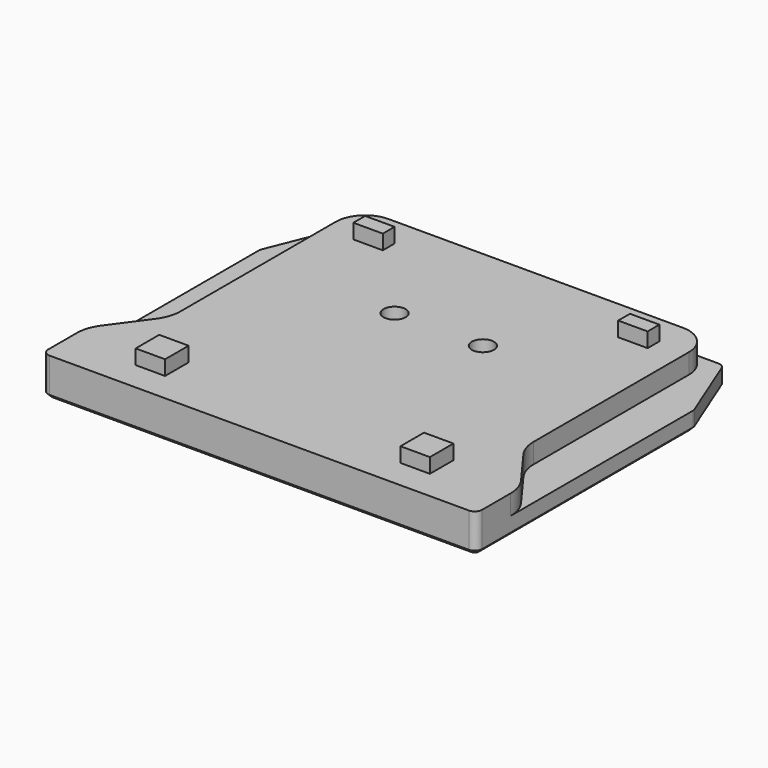
from build123d import *

# Parameters (mm, degrees)
F1_DEPTH      = 2.5
F3_DEPTH      = 2.7
F4_R          = 1
F5_R          = 5
F6_W          = 4
F6_H          = 2
F6_H_2        = 4
F7_DEPTH      = 2
F8_R          = 1.5
F9_DEPTH      = 6
F10_R         = 2.5
F11_DEPTH     = 3.5
F12_S5_R      = 1.5
F12_T6_DEPTH  = 5
F12_S11_R     = 1.5
F12_T12_DEPTH = 5
F13_SIZE      = 0.5


# Not quite as in the source:
# - a fillet or chamfer that OpenCascade refuses, or shapes differently, is made with other operations: its cross-section is extruded or revolved along the edge and cut away or added


with BuildPart() as f1:
    # F0 (on Top) → F1 (new body)
    with BuildSketch(Plane.XY):
        Polygon((55, 0), (4, 0), (0, -10), (0, -47), (59, -47), (59, -10), align=None)
    extrude(amount=F1_DEPTH)

    # F2 (on face) → F3 (join)
    with BuildSketch(Plane.XY.offset(2.5)):
        with BuildLine():
            Line((0, -39.5), (0, -47))
            Line((0, -47), (59, -47))
            Line((59, -47), (59, -39.5))
            Line((59, -39.5), (53.5, -32))
            Line((53.5, -32), (53.5, -4))
            ThreePointArc((53.5, -4), (52.3284271247, -1.1715728753), (49.5, 0))
            Line((49.5, 0), (9.5, 0))
            ThreePointArc((9.5, 0), (6.6715728753, -1.1715728753), (5.5, -4))
            Line((5.5, -4), (5.5, -32))
            Line((5.5, -32), (0, -39.5))
        make_face()
    extrude(amount=F3_DEPTH)

    # F4
    f4_edges = [f1.edges().sort_by_distance(p)[0] for p in [
        (0, -47, 2.6),
        (59, -47, 2.6),
        (4, 0, 1.25),
        (55, 0, 1.25),
        (59, -10, 1.25),
        (0, -10, 1.25),
    ]]
    fillet(f4_edges, radius=F4_R)

    # F5
    f5_edges = [f1.edges().sort_by_distance(p)[0] for p in [
        (0, -39.5, 3.85),
        (59, -39.5, 3.85),
        (53.5, -32, 3.85),
        (5.5, -32, 3.85),
    ]]
    fillet(f5_edges, radius=F5_R)

    # F6 (on face) → F7 (join)
    with BuildSketch(Plane.XY.offset(5.2)):
        with Locations((11.5, -5)):
            Rectangle(F6_W, F6_H)
        with Locations((11.5, -41)):
            Rectangle(F6_W, F6_H_2)
        with Locations((47.5, -5)):
            Rectangle(F6_W, F6_H)
        with Locations((47.5, -41)):
            Rectangle(F6_W, F6_H_2)
    extrude(amount=F7_DEPTH)

    # F8 (on face) → F9 (cut)
    with BuildSketch(Plane.XY.offset(5.2)):
        with Locations((23.5, -16.5)):
            Circle(F8_R)
        with Locations((35.5, -16.5)):
            Circle(F8_R)
    extrude(amount=-F9_DEPTH, mode=Mode.SUBTRACT)

    # F10 (on face) → F11 (cut)
    with BuildSketch(Plane.XY):
        with Locations((35.5, -16.5)):
            Circle(F10_R)
        with Locations((23.5, -16.5)):
            Circle(F10_R)
    extrude(amount=F11_DEPTH, mode=Mode.SUBTRACT)

    # F12: chamfer of 1.2 on 2 edges, made by hand


with BuildPart() as f12_tool2:
    # F12_s3 → F12_t4 (revolve)
    with BuildSketch(Plane.XZ.offset(16.5)):
        Polygon((38, 2.3), (36.8, 3.5), (38, 3.5), align=None)
    revolve(axis=Axis((35.5, -16.5, 3.5), (0, 0, 1)))

    # F12_s5 → F12_t6 (cut, symmetric)
    with BuildSketch(Plane.XY.offset(2.9)):
        with Locations((35.5, -16.5)):
            Circle(F12_S5_R)
    extrude(amount=F12_T6_DEPTH, both=True, mode=Mode.SUBTRACT)


with BuildPart() as f1_1:
    add(f1.part)

    # F12_t1: union F12_tool2
    add(f12_tool2.part)


with BuildPart() as f12_tool8:
    # F12_s9 → F12_t10 (revolve)
    with BuildSketch(Plane.XZ.offset(16.5)):
        Polygon((26, 2.3), (24.8, 3.5), (26, 3.5), align=None)
    revolve(axis=Axis((23.5, -16.5, 3.5), (0, 0, 1)))

    # F12_s11 → F12_t12 (cut, symmetric)
    with BuildSketch(Plane.XY.offset(2.9)):
        with Locations((23.5, -16.5)):
            Circle(F12_S11_R)
    extrude(amount=F12_T12_DEPTH, both=True, mode=Mode.SUBTRACT)


with BuildPart() as f1_2:
    add(f1_1.part)

    # F12_t7: union F12_tool8
    add(f12_tool8.part)

    # F13
    f13_edges = [f1_2.edges().sort_by_distance(p)[0] for p in [
        (29.5, 0, 0),
        (54.883596, -0.171933, 0),
        (4.116404, -0.171933, 0),
        (57.08996, -5.224901, 0),
        (1.91004, -5.224901, 0),
        (58.981956, -10.003475, 0),
        (0.018044, -10.003475, 0),
        (59, -28.096291, 0),
        (0, -28.096291, 0),
        (58.707107, -46.707107, 0),
        (0.292893, -46.707107, 0),
        (29.5, -47, 0),
        (21, -16.5, 0),
        (33, -16.5, 0),
    ]]
    chamfer(f13_edges, length=F13_SIZE)


solid = f1_2.part
